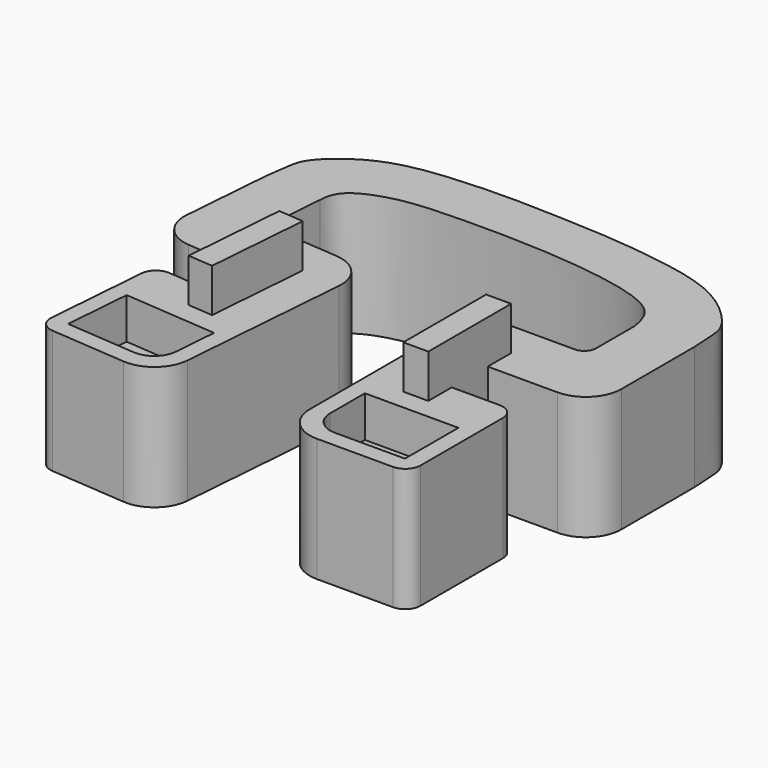
from build123d import *

# Parameters (mm, degrees)
F1_DEPTH      = 9.398
F3_DEPTH      = 3.1242
F5_DEPTH      = 3.1242
F7_DEPTH      = 3.302
F10_R         = 1.7737881333
F10_TEXT_SIZE = 7.1809698258
F11_DEPTH     = 3.81


# Not quite as in the source:
# - Text() gives the source's letters only with a copy of the font that has no kerning and outlines rounded to 1/6400 em; it was checked with that copy


with BuildPart() as f1:
    # F0 (on Top) → F1 (new body)
    with BuildSketch(Plane.XY):
        with BuildLine():
            ThreePointArc((0, -15.8479231639), (0.7890768363, -17.7529231637), (2.6940768361, -18.542))
            Line((2.6940768361, -18.542), (8.4845667062, -18.542))
            ThreePointArc((8.4845667062, -18.542), (9.3100667048, -18.2000667048), (9.652, -17.3745667062))
            Line((9.652, -17.3745667062), (9.652, -9.5494332938))
            ThreePointArc((9.652, -9.5494332938), (9.3100667048, -8.7239332952), (8.4845667062, -8.382))
            Line((8.4845667062, -8.382), (4.826, -8.382))
            Line((4.826, -8.382), (4.826, -4.953))
            Line((4.826, -4.953), (10.1329231639, -4.953))
            ThreePointArc((10.1329231639, -4.953), (12.0379231637, -4.1639231637), (12.827, -2.2589231639))
            Line((12.827, -2.2589231639), (12.827, 4.699))
            add(Edge.make_bspline(
                [(12.827, 4.699), (12.6632187365, 6.5137696787), (12.9781512544, 7.5227069279), (9.4121636869, 11.1637159169), (3.2451314589, 12.2395701223), (0, 12.5623311505), (-3.683, 12.7)],
                knots=[0, 0, 0, 0, 0.1948664127, 0.4240387551, 0.6933385773, 1, 1, 1, 1], degree=3))
            add(Edge.make_bspline(
                [(-20.7698564049, 6.0190240833), (-20.4641948364, 7.8153493028), (-20.6989962183, 8.8458856558), (-16.8583311275, 12.1958864693), (-10.6258992536, 12.7845644033), (-7.3654479136, 12.8517203872), (-3.683, 12.7)],
                knots=[0, 0, 0, 0, 0.1948664127, 0.4240387551, 0.6933385773, 1, 1, 1, 1], degree=3))
            Line((-20.7698564049, 6.0190240833), (-21.3157687644, -0.9174501256))
            ThreePointArc((-21.3157687644, -0.9174501256), (-20.6785889661, -2.8784879012), (-18.8413717005, -3.8145968543))
            Line((-18.8413717005, -3.8145968543), (-13.5508080096, -4.2309732468))
            Line((-13.5508080096, -4.2309732468), (-13.8198442489, -7.6494027842))
            Line((-13.8198442489, -7.6494027842), (-17.4671328149, -7.3623549488))
            ThreePointArc((-17.4671328149, -7.3623549488), (-18.3169158497, -7.6384661943), (-18.722563062, -8.4345936748))
            Line((-18.722563062, -8.4345936748), (-19.3365159535, -16.2356048124))
            ThreePointArc((-19.3365159535, -16.2356048124), (-19.060404708, -17.0853878472), (-18.2642772275, -17.4910350595))
            Line((-18.2642772275, -17.4910350595), (-12.4916375052, -17.9453516585))
            ThreePointArc((-12.4916375052, -17.9453516585), (-10.5305997296, -17.3081718602), (-9.5944907765, -15.4709545946))
            Line((-9.5944907765, -15.4709545946), (-8.5624518883, -2.3576571852))
            ThreePointArc((-8.5624518883, -2.3576571852), (-9.1996316866, -0.3966194095), (-11.0368489522, 0.5394895435))
            Line((-11.0368489522, 0.5394895435), (-15.8119808486, 0.9153005741))
            ThreePointArc((-15.8119808486, 0.9153005741), (-16.4243866037, 1.2273368917), (-16.6367798698, 1.8810161502))
            Line((-16.6367798698, 1.8810161502), (-16.3485231616, 5.5436649014))
            add(Edge.make_bspline(
                [(-16.3485231616, 5.5436649014), (-16.3315940371, 6.2656694879), (-15.8675461895, 7.4947758477), (-12.6168741125, 8.6755627884), (-8.9754333379, 8.8453068611), (-3.7867613646, 8.896328582), (2.697942273, 8.4370235224), (7.6808010629, 7.134305193), (8.2200181522, 5.5049010457), (8.382, 4.572)],
                knots=[0, 0, 0, 0, 0.0992930418, 0.2292969548, 0.3703348189, 0.5371197124, 0.7286259605, 0.887182054, 1, 1, 1, 1], degree=3))
            Line((8.382, 4.572), (8.382, 0.8980256119))
            ThreePointArc((8.382, 0.8980256119), (8.118974388, 0.263025612), (7.4839743881, 0))
            Line((7.4839743881, 0), (2.6940768361, 0))
            ThreePointArc((2.6940768361, 0), (0.7890768363, -0.7890768363), (0, -2.6940768361))
            Line((0, -2.6940768361), (0, -15.8479231639))
        make_face()
    extrude(amount=F1_DEPTH)

    # F2 (on face) → F3 (cut)
    with BuildSketch(Plane.XY.offset(9.398)):
        with BuildLine():
            Line((-10.8328072989, -15.0184794061), (-10.7189954805, -13.5723631399))
            Line((-10.7189954805, -13.5723631399), (-10.5737353648, -11.7266583701))
            Line((-10.5737353648, -11.7266583701), (-17.6638114423, -11.1686572813))
            Line((-17.6638114423, -11.1686572813), (-18.0623836486, -16.2329973367))
            Line((-18.0623836486, -16.2329973367), (-12.7448265905, -16.6514981533))
            ThreePointArc((-12.7448265905, -16.6514981533), (-11.4506076884, -16.2309809408), (-10.8328072989, -15.0184794061))
        make_face()
        with BuildLine():
            Line((1.27, -12.192), (1.27, -14.0434120553))
            Line((1.27, -14.0434120553), (1.27, -15.494))
            ThreePointArc((1.27, -15.494), (1.7907641431, -16.7512358569), (3.048, -17.272))
            Line((3.048, -17.272), (8.382, -17.272))
            Line((8.382, -17.272), (8.382, -12.192))
            Line((8.382, -12.192), (1.27, -12.192))
        make_face()
    extrude(amount=-F3_DEPTH, mode=Mode.SUBTRACT)

    # F4 (on face) → F5 (cut)
    with BuildSketch(Plane(origin=(0, 0, 0), x_dir=(1, 0, 0), z_dir=(0, 0, -1))):
        with BuildLine():
            Line((8.382, 9.652), (8.382, 17.272))
            Line((8.382, 17.272), (3.048, 17.272))
            ThreePointArc((3.048, 17.272), (1.7907641431, 16.7512358569), (1.27, 15.494))
            Line((1.27, 15.494), (1.27, 9.652))
            Line((1.27, 9.652), (8.382, 9.652))
        make_face()
        with BuildLine():
            Line((-12.7448265905, 16.6514981533), (-18.0623836486, 16.2329973367))
            Line((-18.0623836486, 16.2329973367), (-17.4645253392, 8.6364872536))
            Line((-17.4645253392, 8.6364872536), (-10.3744492617, 9.1944883425))
            Line((-10.3744492617, 9.1944883425), (-10.8328072989, 15.0184794061))
            ThreePointArc((-10.8328072989, 15.0184794061), (-11.4506076884, 16.2309809408), (-12.7448265905, 16.6514981533))
        make_face()
    extrude(amount=-F5_DEPTH, mode=Mode.SUBTRACT)

    # F6 (on face) → F7 (join)
    with BuildSketch(Plane.XY.offset(9.398)):
        Polygon((-13.3764326694, -2.0153244726), (-13.5508080096, -4.2309732468), (-13.8198442489, -7.6494027842), (-13.9942195891, -9.8650515584), (-12.0950920684, -10.0145161358), (-11.4773051486, -2.16478905), align=None)
        Polygon((4.826, -8.382), (4.826, -4.953), (4.826, -2.7305), (2.921, -2.7305), (2.921, -10.6045), (4.826, -10.6045), align=None)
    extrude(amount=F7_DEPTH)

    # F10 (on line) → F11 (cut)
    with BuildSketch(Plane(origin=(0.5784272043, 14.039168306, 0), x_dir=(-0.9991523195, 0.0411660342, 0), z_dir=(0.0411660342, 0.9991523195, 0))):
        with BuildLine():
            Line((-6.1671788015, 7.56964706), (-5.980000163, 7.0864832983))
            ThreePointArc((-5.980000163, 7.0864832983), (-6.1928696303, 6.9675179327), (-6.3942471449, 6.8299924262))
            Line((-6.3942471449, 6.8299924262), (-6.7433249095, 7.212912493))
            Line((-6.7433249095, 7.212912493), (-7.1262449763, 6.8638347283))
            Line((-7.1262449763, 6.8638347283), (-6.7771672117, 6.4809146615))
            ThreePointArc((-6.7771672117, 6.4809146615), (-6.9326868315, 6.2930854408), (-7.0707858284, 6.0921007762))
            Line((-7.0707858284, 6.0921007762), (-7.5346178328, 6.3230616713))
            Line((-7.5346178328, 6.3230616713), (-7.7655787278, 5.8592296669))
            Line((-7.7655787278, 5.8592296669), (-7.3017467234, 5.6282687719))
            ThreePointArc((-7.3017467234, 5.6282687719), (-7.3789127094, 5.396943073), (-7.4350821538, 5.1596433431))
            Line((-7.4350821538, 5.1596433431), (-7.9510253155, 5.2074525177))
            Line((-7.9510253155, 5.2074525177), (-7.9988344902, 4.691509356))
            Line((-7.9988344902, 4.691509356), (-7.4828913284, 4.6437001813))
            ThreePointArc((-7.4828913284, 4.6437001813), (-7.4712819865, 4.4001198219), (-7.4379358837, 4.15855367))
            Line((-7.4379358837, 4.15855367), (-7.9363092199, 4.0167542303))
            Line((-7.9363092199, 4.0167542303), (-7.7945097801, 3.5183808941))
            Line((-7.7945097801, 3.5183808941), (-7.2961364439, 3.6601803338))
            ThreePointArc((-7.2961364439, 3.6601803338), (-7.1973196801, 3.4372421911), (-7.0789616061, 3.2240344646))
            Line((-7.0789616061, 3.2240344646), (-7.4924570361, 2.9117772105))
            Line((-7.4924570361, 2.9117772105), (-7.180199782, 2.4982817805))
            Line((-7.180199782, 2.4982817805), (-6.766704352, 2.8105390346))
            ThreePointArc((-6.766704352, 2.8105390346), (-6.5940259178, 2.63835214), (-6.4066407863, 2.4822977238))
            Line((-6.4066407863, 2.4822977238), (-6.679413461, 2.0417547279))
            Line((-6.679413461, 2.0417547279), (-6.2388704651, 1.7689820532))
            Line((-6.2388704651, 1.7689820532), (-5.9660977904, 2.2095250491))
            ThreePointArc((-5.9660977904, 2.2095250491), (-5.7428788651, 2.1113441969), (-5.5117740765, 2.0335191047))
            Line((-5.5117740765, 2.0335191047), (-5.6069845347, 1.5241881396))
            Line((-5.6069845347, 1.5241881396), (-5.0976535696, 1.4289776814))
            Line((-5.0976535696, 1.4289776814), (-5.0024431114, 1.9383086465))
            ThreePointArc((-5.0024431114, 1.9383086465), (-4.7588306479, 1.9273937048), (-4.5152181844, 1.9383086465))
            Line((-4.5152181844, 1.9383086465), (-4.4200077262, 1.4289776814))
            Line((-4.4200077262, 1.4289776814), (-3.9106767611, 1.5241881396))
            Line((-3.9106767611, 1.5241881396), (-4.0058872194, 2.0335191047))
            ThreePointArc((-4.0058872194, 2.0335191047), (-3.7747824307, 2.1113441969), (-3.5515635055, 2.2095250491))
            Line((-3.5515635055, 2.2095250491), (-3.2787908308, 1.7689820532))
            Line((-3.2787908308, 1.7689820532), (-2.8382478348, 2.0417547279))
            Line((-2.8382478348, 2.0417547279), (-3.1110205095, 2.4822977238))
            ThreePointArc((-3.1110205095, 2.4822977238), (-2.923635378, 2.63835214), (-2.7509569438, 2.8105390346))
            Line((-2.7509569438, 2.8105390346), (-2.3374615138, 2.4982817805))
            Line((-2.3374615138, 2.4982817805), (-2.0252042598, 2.9117772105))
            Line((-2.0252042598, 2.9117772105), (-2.4386996897, 3.2240344646))
            ThreePointArc((-2.4386996897, 3.2240344646), (-2.3203416157, 3.4372421911), (-2.2215248519, 3.6601803338))
            Line((-2.2215248519, 3.6601803338), (-1.7231515157, 3.5183808941))
            Line((-1.7231515157, 3.5183808941), (-1.5813520759, 4.0167542303))
            Line((-1.5813520759, 4.0167542303), (-2.0797254121, 4.15855367))
            ThreePointArc((-2.0797254121, 4.15855367), (-2.0463793094, 4.4001198219), (-2.0347699674, 4.6437001813))
            Line((-2.0347699674, 4.6437001813), (-1.5188268057, 4.691509356))
            Line((-1.5188268057, 4.691509356), (-1.5666359803, 5.2074525177))
            Line((-1.5666359803, 5.2074525177), (-2.0825791421, 5.1596433431))
            ThreePointArc((-2.0825791421, 5.1596433431), (-2.1387485865, 5.396943073), (-2.2159145724, 5.6282687719))
            Line((-2.2159145724, 5.6282687719), (-1.752082568, 5.8592296669))
            Line((-1.752082568, 5.8592296669), (-1.9830434631, 6.3230616713))
            Line((-1.9830434631, 6.3230616713), (-2.4468754675, 6.0921007762))
            ThreePointArc((-2.4468754675, 6.0921007762), (-2.5849744643, 6.2930854408), (-2.7404940842, 6.4809146615))
            Line((-2.7404940842, 6.4809146615), (-2.3914163195, 6.8638347283))
            Line((-2.3914163195, 6.8638347283), (-2.7743363863, 7.212912493))
            Line((-2.7743363863, 7.212912493), (-3.123414151, 6.8299924262))
            ThreePointArc((-3.123414151, 6.8299924262), (-3.3247916656, 6.9675179327), (-3.5376611328, 7.0864832983))
            Line((-3.5376611328, 7.0864832983), (-3.3504824944, 7.56964706))
            Line((-3.3504824944, 7.56964706), (-3.8336462561, 7.7568256985))
            Line((-3.8336462561, 7.7568256985), (-4.0208248946, 7.2736619368))
            ThreePointArc((-4.0208248946, 7.2736619368), (-4.2582837776, 7.3291547035), (-4.4997538913, 7.3631892822))
            Line((-4.4997538913, 7.3631892822), (-4.4997538913, 7.8813427955))
            Line((-4.4997538913, 7.8813427955), (-5.0179074046, 7.8813427955))
            Line((-5.0179074046, 7.8813427955), (-5.0179074046, 7.3631892822))
            ThreePointArc((-5.0179074046, 7.3631892822), (-5.2593775182, 7.3291547035), (-5.4968364013, 7.2736619368))
            Line((-5.4968364013, 7.2736619368), (-5.6840150398, 7.7568256985))
            Line((-5.6840150398, 7.7568256985), (-6.1671788015, 7.56964706))
        make_face()
        with Locations((-4.7588306479, 4.6514654532)):
            Circle(F10_R, mode=Mode.SUBTRACT)
        with Locations((-0.6676292978, 1.992772799)):
            Text('MBA', F10_TEXT_SIZE, font='Open Sans', font_style=FontStyle.BOLD, text_align=(TextAlign.LEFT, TextAlign.BOTTOM))
    extrude(amount=-F11_DEPTH, mode=Mode.SUBTRACT)


solid = f1.part
